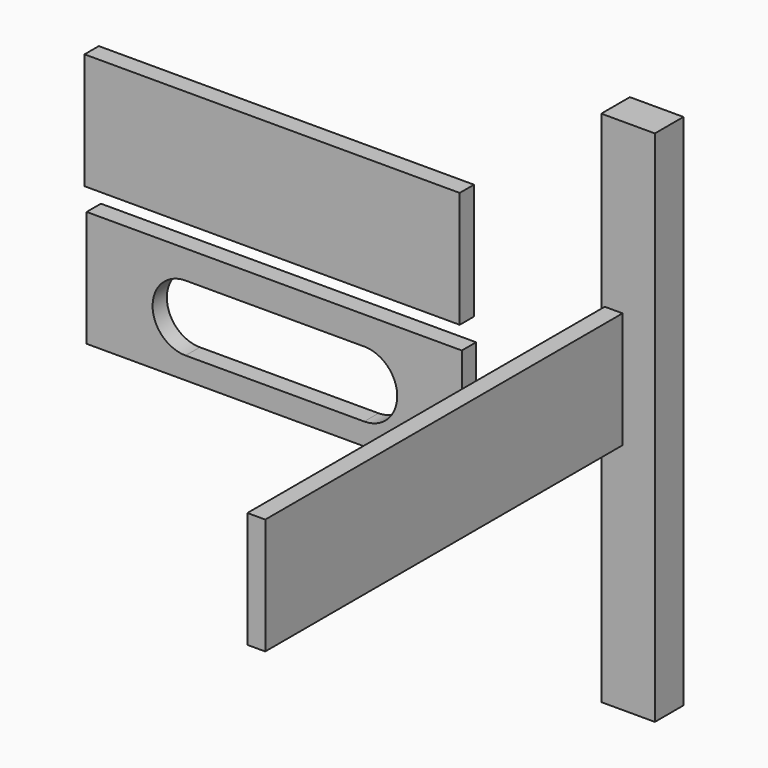
from build123d import *

# Parameters (mm, degrees)
F0_W     = 38.1
F0_H     = 368.3
F1_DEPTH = 25.4
F2_W     = 266.7
F2_H     = 82.55
F3_DEPTH = 12.7
F4_W     = 266.7
F4_H     = 82.55
F5_DEPTH = 12.7
F6_W     = 317.5
F6_H     = 82.55
F7_DEPTH = 12.7


with BuildPart() as f1:
    # F0 (on Front) → F1 (new body)
    with BuildSketch(Plane.XZ):
        Rectangle(F0_W, F0_H)
    extrude(amount=F1_DEPTH)


with BuildPart() as f3:
    # F2 (on Front) → F3 (new body)
    with BuildSketch(Plane.XZ):
        with Locations((-263.197883749, 52.0507570222)):
            Rectangle(F2_W, F2_H)
    extrude(amount=F3_DEPTH)


with BuildPart() as f5:
    # F4 (on Front) → F5 (new body)
    with BuildSketch(Plane.XZ):
        with Locations((-261.7122530937, -46.0856069893)):
            Rectangle(F4_W, F4_H)
        with BuildLine():
            ThreePointArc((-324.7247487307, -71.793478018), (-348.1777791041, -47.9326123349), (-323.9161690893, -24.8943870487))
            Line((-323.9161690893, -24.8943870487), (-196.9161690893, -24.8943870487))
            ThreePointArc((-196.9161690893, -24.8943870487), (-174.2717183572, -48.741312141), (-197.7247487307, -71.793478018))
            Line((-197.7247487307, -71.793478018), (-324.7247487307, -71.793478018))
        make_face(mode=Mode.SUBTRACT)
    extrude(amount=F5_DEPTH)


with BuildPart() as f7:
    # F6 (on Right) → F7 (new body)
    with BuildSketch(Plane.YZ):
        with Locations((-204.9318166077, 36.656818153)):
            Rectangle(F6_W, F6_H)
    extrude(amount=F7_DEPTH)


solid = Compound([f1.part, f3.part, f5.part, f7.part])
